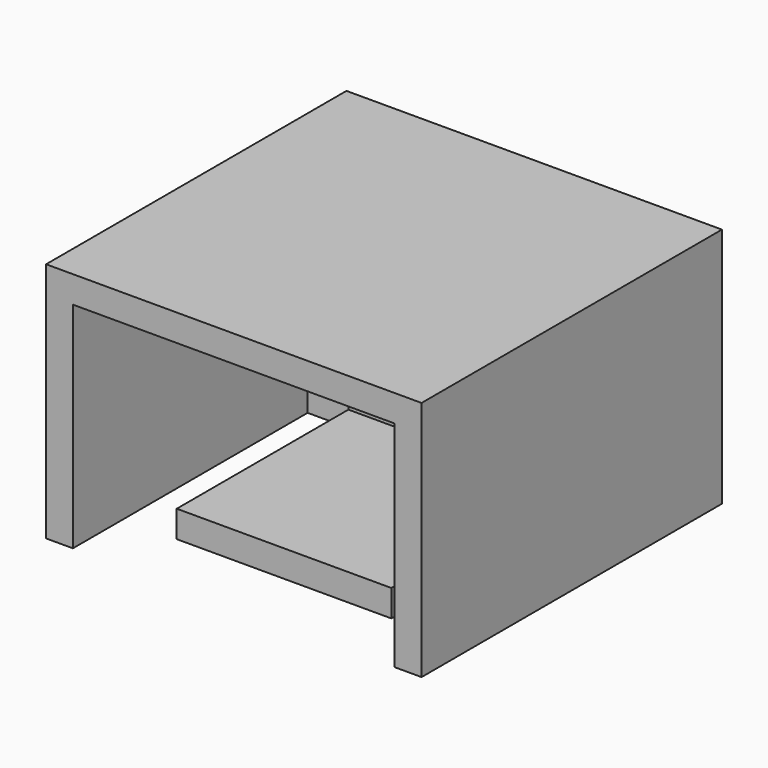
from build123d import *

# Parameters (mm, degrees)
F1_DEPTH = 700
F2_W     = 600
F2_H     = 18
F3_DEPTH = 400
F6_START = 236
F5_R     = 4
F6_DEPTH = 18
F8_DEPTH = 200


# Not quite as in the source:
# - a pattern or mirror of a feature is missing from the dataset's text; its kind, count and spacing are read off the source's solid


with BuildPart() as f1:
    # F0 (on Front) → F1 (new body)
    with BuildSketch(Plane.XZ):
        Polygon((-350, 0), (-300, 0), (-300, 400), (300, 400), (300, 0), (350, 0), (350, 450), (-350, 450), align=None)
    extrude(amount=F1_DEPTH)

    # F2 (on face) → F3 (join)
    with BuildSketch(Plane(origin=(0, 0, 400), x_dir=(1, 0, 0), z_dir=(0, 0, -1))):
        with Locations((0, 144)):
            Rectangle(F2_W, F2_H)
    extrude(amount=F3_DEPTH)

    # F5 (on Right) → F6 (join)
    with BuildSketch(Plane.YZ.offset(F6_START)):
        Polygon((-135, 150), (-135, 0), (-25, 0), (-25, 80), align=None)
        with Locations((-45, 30)):
            Circle(F5_R, mode=Mode.SUBTRACT)
    f6 = extrude(amount=F6_DEPTH)

    # F6_copies: F6 across plane
    add(f6.mirror(Plane(origin=(0, 0, 0), x_dir=(0, 0, -1), z_dir=(-1, 0, 0))))

    # F7 (on Right) → F8 (join, symmetric)
    with BuildSketch(Plane.YZ):
        Polygon((-583, 50), (-583, 0), (-153, 0), (-153, 350), (-183, 350), (-183, 50), align=None)
    extrude(amount=F8_DEPTH, both=True)


solid = f1.part
